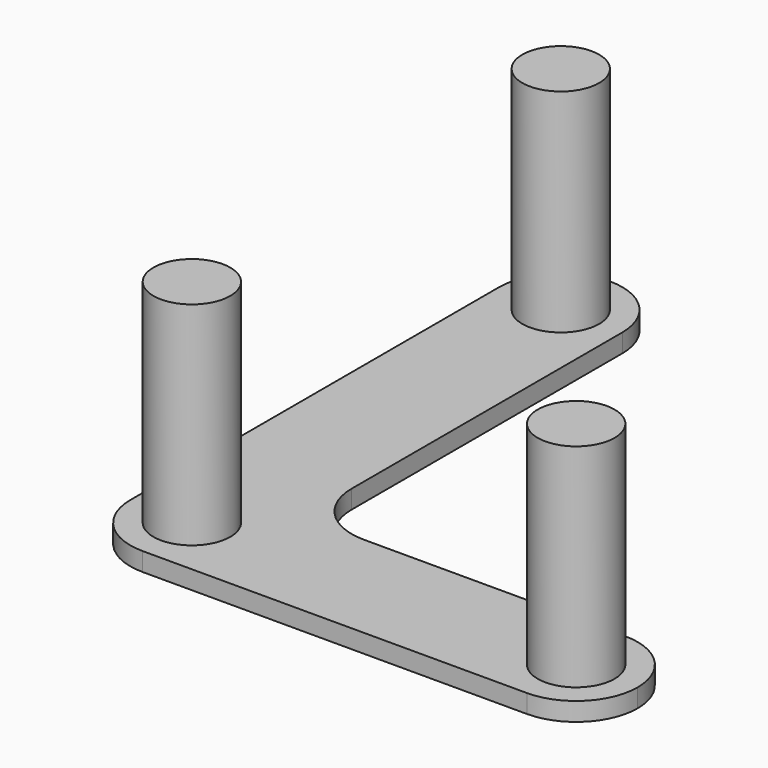
from build123d import *

# Parameters (mm, degrees)
F0_R     = 2.5
F1_DEPTH = 1.2
F2_DEPTH = 15
F3_R     = 3.99999


# Not quite as in the source:
# - a fillet or chamfer is up to 0.001 mm smaller than in the source, because OpenCascade refuses the exact size


with BuildPart() as f1:
    # F0 (on Top) → F1 (new body)
    with BuildSketch(Plane.XY):
        Polygon((4, 34), (-4, 34), (-4, -4), (29, -4), (29, 4), (4, 4), align=None)
        Circle(F0_R, mode=Mode.SUBTRACT)
        with Locations((25, 0)):
            Circle(F0_R, mode=Mode.SUBTRACT)
        with Locations((0, 30)):
            Circle(F0_R, mode=Mode.SUBTRACT)
    extrude(amount=F1_DEPTH)

    # F0 (on Top) → F2 (join)
    with BuildSketch(Plane.XY):
        Circle(F0_R)
        with Locations((25, 0)):
            Circle(F0_R)
        with Locations((0, 30)):
            Circle(F0_R)
    extrude(amount=F2_DEPTH)

    # F3 (radius 4 in the source; OpenCascade refuses exactly that, so slightly less here)
    f3_edges = [f1.edges().sort_by_distance(p)[0] for p in [
        (4, 4, 0.6),
        (29, 4, 0.6),
        (29, -4, 0.6),
        (-4, -4, 0.6),
        (-4, 34, 0.6),
        (4, 34, 0.6),
    ]]
    fillet(f3_edges, radius=F3_R)


solid = f1.part
